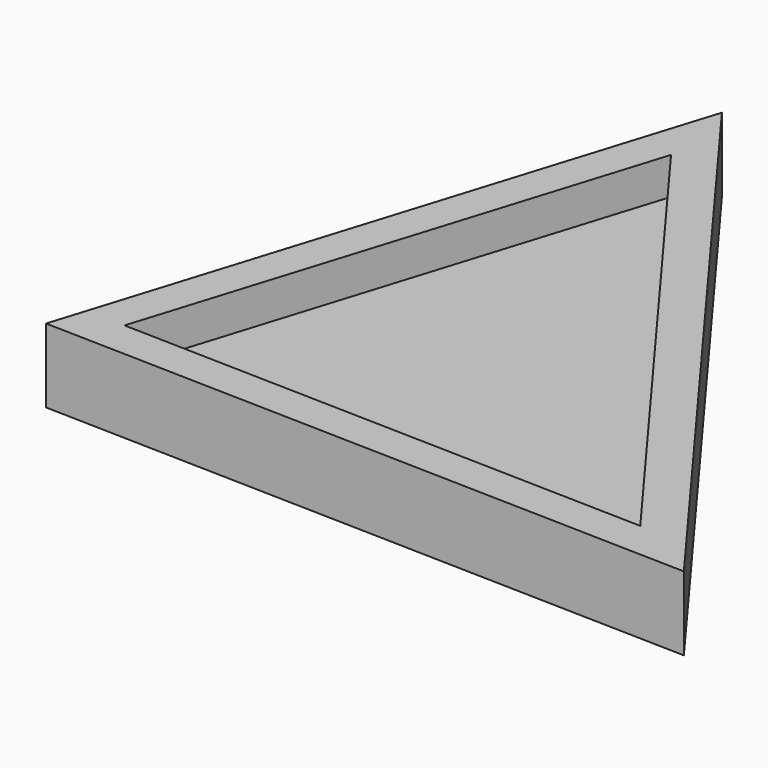
from build123d import *

# Parameters (mm, degrees)
F1_DEPTH = 6.35
F3_T     = 6.35


# Not quite as in the source:
# - a feature names something its author has since deleted; it is built from what else it names


with BuildPart() as f1:
    # F0 (on Top) → F1 (new body)
    with BuildSketch(Plane.XY):
        Polygon((-47.7481111884, 27.6977252215), (-74.0418732166, -56.7705929279), (16.344493255, -59.0262524784), align=None)
    extrude(amount=F1_DEPTH)

    # F3
    f3_openings = [f1.faces().sort_by_distance(p)[0] for p in [
        (-35.148497, -29.366373, 6.35),
    ]]
    offset(amount=F3_T, openings=f3_openings, kind=Kind.INTERSECTION)


solid = f1.part
